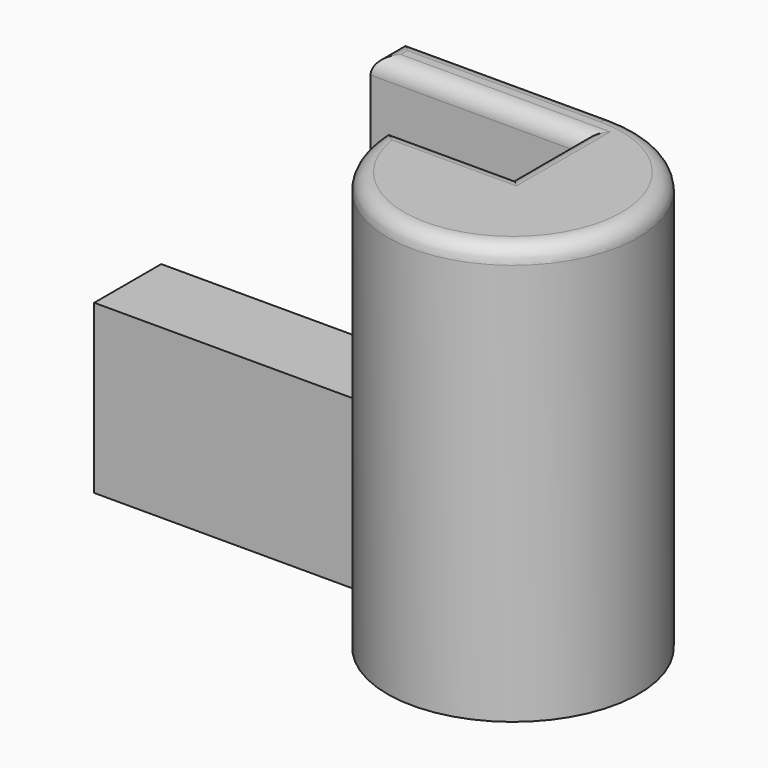
from build123d import *

# Parameters (mm, degrees)
F0_W     = 12.5
F0_H     = 2.5
F1_DEPTH = 25
F2_R     = 1
F3_DEPTH = 10


with BuildPart() as f1:
    # F0 (on Top) → F1 (new body)
    with BuildSketch(Plane.XY):
        with BuildLine():
            Line((0, 7.5), (0, 5))
            Line((0, 5), (0, 0))
            Line((0, 0), (-7.5, 0))
            ThreePointArc((-7.5, 0), (0, -7.5), (7.5, 0))
            ThreePointArc((7.5, 0), (5.3033008589, 5.3033008589), (0, 7.5))
        make_face()
        with Locations((-6.25, 6.25)):
            Rectangle(F0_W, F0_H)
    extrude(amount=F1_DEPTH)

    # F2
    f2_edges = [f1.edges().sort_by_distance(p)[0] for p in [
        (-6.25, 7.5, 25),
        (-12.5, 6.25, 25),
        (-6.25, 5, 25),
        (0, 2.5, 25),
        (-3.75, 0, 25),
        (5.303301, -5.303301, 25),
    ]]
    fillet(f2_edges, radius=F2_R)

    # F0 (on Top) → F3 (join)
    with BuildSketch(Plane.XY):
        Polygon((0, 5), (-12.5, 5), (-12.5, 0), (-7.5, 0), (0, 0), align=None)
        with BuildLine():
            Line((-12.5, 0), (-12.5, 5))
            ThreePointArc((-12.5, 5), (-16.0355339059, 3.5355339059), (-17.5, 0))
            Line((-17.5, 0), (-12.5, 0))
        make_face()
        with BuildLine():
            ThreePointArc((-17.5, 0), (-16.0355339059, 3.5355339059), (-12.5, 5))
            Line((-12.5, 5), (-25, 5))
            Line((-25, 5), (-25, 0))
            Line((-25, 0), (-17.5, 0))
        make_face()
    extrude(amount=F3_DEPTH)


solid = f1.part
